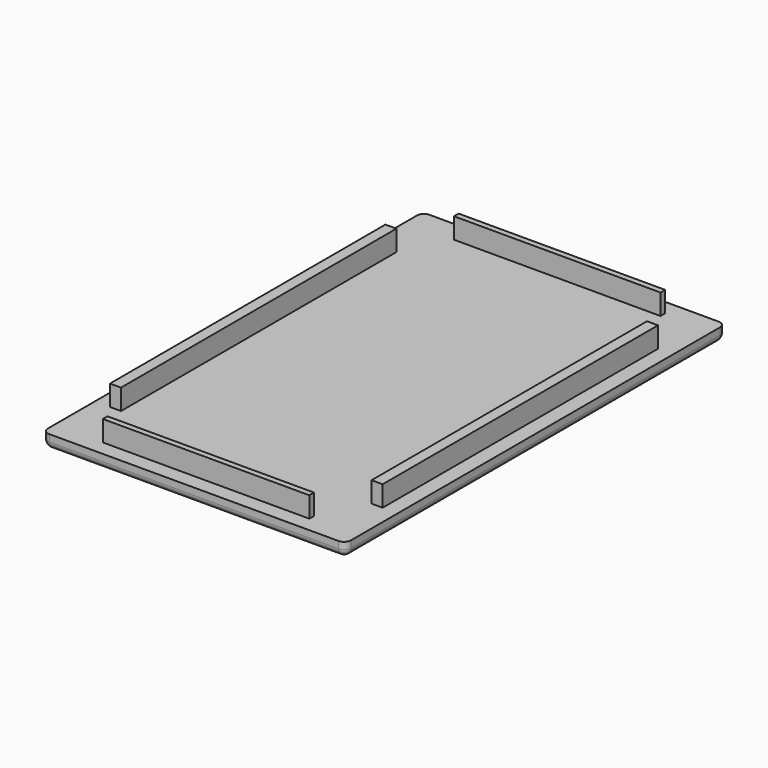
from build123d import *

# Parameters (mm, degrees)
F0_W     = 30
F0_H     = 0.843597576
F0_W_2   = 1.6
F0_H_2   = 50
F1_DEPTH = 2
F2_DEPTH = 5
F3_R     = 1


with BuildPart() as f1:
    # F0 (on Top) → F1 (new body)
    with BuildSketch(Plane.XY):
        with BuildLine():
            Line((-19, -34.5), (23, -34.5))
            ThreePointArc((23, -34.5), (23.7071067812, -34.2071067812), (24, -33.5))
            Line((24, -33.5), (24, 33.5))
            ThreePointArc((24, 33.5), (23.7071067812, 34.2071067812), (23, 34.5))
            Line((23, 34.5), (-19, 34.5))
            ThreePointArc((-19, 34.5), (-19.7071067812, 34.2071067812), (-20, 33.5))
            Line((-20, 33.5), (-20, -33.5))
            ThreePointArc((-20, -33.5), (-19.7071067812, -34.2071067812), (-19, -34.5))
        make_face()
        with Locations((2, -31.878201212)):
            Rectangle(F0_W, F0_H, mode=Mode.SUBTRACT)
        with Locations((-17, 0)):
            Rectangle(F0_W_2, F0_H_2, mode=Mode.SUBTRACT)
        with Locations((21, 0)):
            Rectangle(F0_W_2, F0_H_2, mode=Mode.SUBTRACT)
        with Locations((2, 31.878201212)):
            Rectangle(F0_W, F0_H, mode=Mode.SUBTRACT)
    extrude(amount=F1_DEPTH)

    # F0 (on Top) → F2 (join)
    with BuildSketch(Plane.XY):
        with Locations((-17, 0)):
            Rectangle(F0_W_2, F0_H_2)
        with Locations((2, 31.878201212)):
            Rectangle(F0_W, F0_H)
        with Locations((21, 0)):
            Rectangle(F0_W_2, F0_H_2)
        with Locations((2, -31.878201212)):
            Rectangle(F0_W, F0_H)
    extrude(amount=F2_DEPTH)

    # F3
    f3_edges = [f1.edges().sort_by_distance(p)[0] for p in [
        (-20, 0, 0),
        (-19.707107, -34.207107, 0),
        (2, -34.5, 0),
        (23.707107, -34.207107, 0),
        (24, 0, 0),
        (23.707107, 34.207107, 0),
        (2, 34.5, 0),
        (-19.707107, 34.207107, 0),
    ]]
    fillet(f3_edges, radius=F3_R)


solid = f1.part
